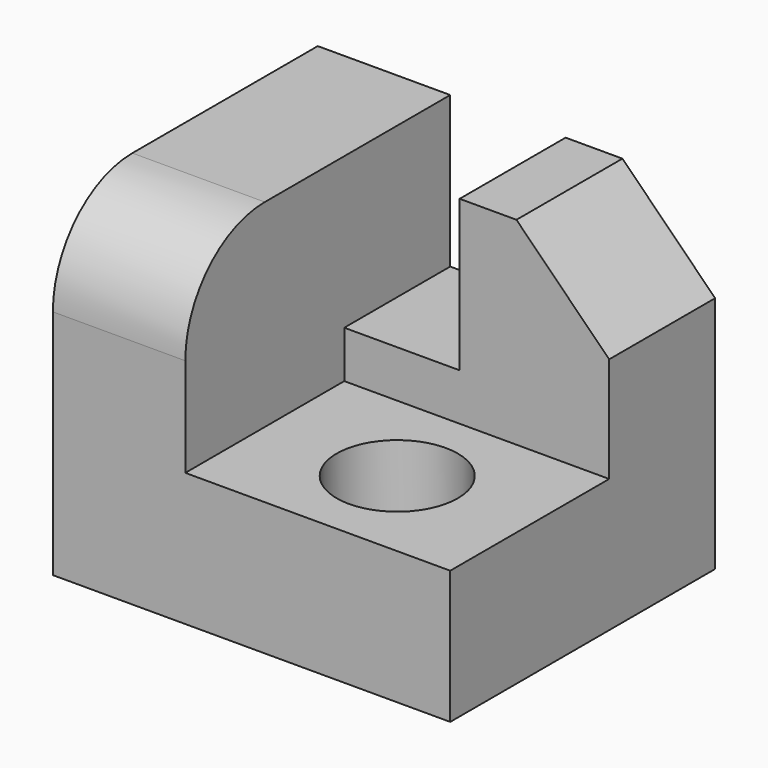
from build123d import *

# Parameters (mm, degrees)
F0_W     = 152.4
F0_H     = 127
F1_DEPTH = 127
F2_W     = 101.6
F2_H     = 76.2
F3_DEPTH = 75.946
F4_R     = 23.2368410965
F5_DEPTH = 177.8
F6_R     = 38.1
F7_SIZE  = 35.56
F8_W     = 44.2467968255
F8_H     = 50.8
F9_DEPTH = 57.912


# Not quite as in the source:
# - a feature names something its author has since deleted; it is built from what else it names


with BuildPart() as f1:
    # F0 (on Front) → F1 (new body)
    with BuildSketch(Plane.XZ):
        Rectangle(F0_W, F0_H)
    extrude(amount=F1_DEPTH)

    # F2 (on face) → F3 (cut)
    with BuildSketch(Plane.XY.offset(63.5)):
        with Locations((25.4, -88.9)):
            Rectangle(F2_W, F2_H)
    extrude(amount=-F3_DEPTH, mode=Mode.SUBTRACT)

    # F4 (on face) → F5 (cut)
    with BuildSketch(Plane.XY.offset(-12.446)):
        with Locations((25.4, -88.9)):
            Circle(F4_R)
    extrude(amount=-F5_DEPTH, mode=Mode.SUBTRACT)

    # F6
    f6_edges = [f1.edges().sort_by_distance(p)[0] for p in [
        (-50.8, -127, 63.5),
    ]]
    fillet(f6_edges, radius=F6_R)

    # F7
    f7_edges = [f1.edges().sort_by_distance(p)[0] for p in [
        (76.2, -25.4, 63.5),
    ]]
    chamfer(f7_edges, length=F7_SIZE)

    # F8 (on face) → F9 (cut)
    with BuildSketch(Plane.XY.offset(63.5)):
        with Locations((-3.2766015872, -25.4)):
            Rectangle(F8_W, F8_H)
    extrude(amount=-F9_DEPTH, mode=Mode.SUBTRACT)


solid = f1.part
